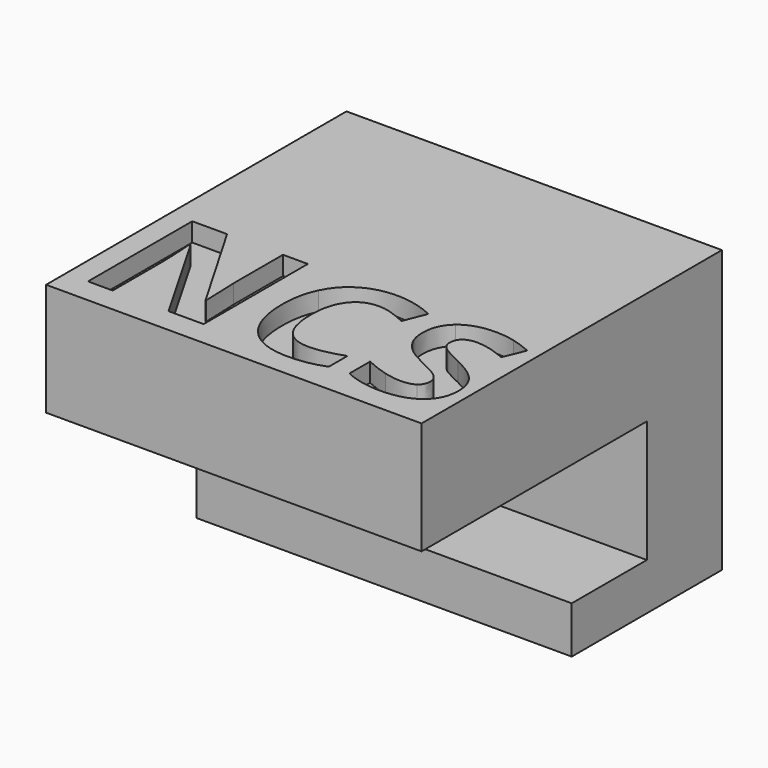
from build123d import *

# Parameters (mm, degrees)
F0_W         = 40
F0_H         = 10
F1_DEPTH     = 5
F2_DEPTH     = 13
F3_START     = 13
F0_H_2       = 20
F3_DEPTH     = 12
F4_START     = 13
F0_TEXT_SIZE = 19.4444444444
F4_DEPTH     = 10


# Not quite as in the source:
# - Text() gives the source's letters only with a copy of the font that has no kerning and outlines rounded to 1/6400 em; it was checked with that copy


with BuildPart() as f1:
    # F0 (on Top) → F1 (new body)
    with BuildSketch(Plane.XY):
        with Locations((0, 15)):
            Rectangle(F0_W, F0_H)
        with Locations((0, 5)):
            Rectangle(F0_W, F0_H)
    extrude(amount=-F1_DEPTH)

    # F0 (on Top) → F2 (join)
    with BuildSketch(Plane.XY):
        with Locations((0, 15)):
            Rectangle(F0_W, F0_H)
    extrude(amount=F2_DEPTH)

    # F0 (on Top) → F3 (join)
    with BuildSketch(Plane.XY.offset(F3_START)):
        with Locations((0, -10)):
            Rectangle(F0_W, F0_H_2)
        with BuildLine():
            Line((-5.3385416667, -3.4717519035), (-5.3385416667, -17.3532623202))
            Line((-5.3385416667, -17.3532623202), (-9.0785590278, -17.3532623202))
            Line((-9.0785590278, -17.3532623202), (-15.1184895833, -6.8532623202))
            Line((-15.1184895833, -6.8532623202), (-15.2035590278, -6.8532623202))
            add(Edge.make_bspline(
                [(-15.2035590278, -6.8532623202), (-15.0212673611, -9.6332102368), (-15.0212673611, -10.8211442646)],
                knots=[0, 0, 0, 1, 1, 1], degree=2))
            Line((-15.0212673611, -10.8211442646), (-15.0212673611, -17.3532623202))
            Line((-15.0212673611, -17.3532623202), (-17.65234375, -17.3532623202))
            Line((-17.65234375, -17.3532623202), (-17.65234375, -3.4717519035))
            Line((-17.65234375, -3.4717519035), (-13.9396701389, -3.4717519035))
            Line((-13.9396701389, -3.4717519035), (-7.9118923611, -13.8684532924))
            Line((-7.9118923611, -13.8684532924), (-7.8450520833, -13.8684532924))
            add(Edge.make_bspline(
                [(-7.8450520833, -13.8684532924), (-7.9878472222, -11.1614220424), (-7.9878472222, -10.0433664868)],
                knots=[0, 0, 0, 1, 1, 1], degree=2))
            Line((-7.9878472222, -10.0433664868), (-7.9878472222, -3.4717519035))
            Line((-7.9878472222, -3.4717519035), (-5.3385416667, -3.4717519035))
        make_face(mode=Mode.SUBTRACT)
        with BuildLine():
            add(Edge.make_bspline(
                [(5.5989583333, -5.998010584), (4.8120659722, -5.7230539868), (4.0525173611, -5.7230539868)],
                knots=[0, 0, 0, 1, 1, 1], degree=2))
            add(Edge.make_bspline(
                [(4.0525173611, -5.7230539868), (2.390625, -5.7230539868), (1.4791666667, -6.9717519035)],
                knots=[0, 0, 0, 1, 1, 1], degree=2))
            add(Edge.make_bspline(
                [(1.4791666667, -6.9717519035), (0.5677083333, -8.2204498202), (0.5677083333, -10.4504845424)],
                knots=[0, 0, 0, 1, 1, 1], degree=2))
            add(Edge.make_bspline(
                [(0.5677083333, -10.4504845424), (0.5677083333, -15.0928456535), (4.0525173611, -15.0928456535)],
                knots=[0, 0, 0, 1, 1, 1], degree=2))
            add(Edge.make_bspline(
                [(4.0525173611, -15.0928456535), (5.5138888889, -15.0928456535), (7.5920138889, -14.3636789868)],
                knots=[0, 0, 0, 1, 1, 1], degree=2))
            Line((7.5920138889, -14.3636789868), (7.5920138889, -16.8306928757))
            add(Edge.make_bspline(
                [(7.5920138889, -16.8306928757), (5.8845486111, -17.5446685702), (3.7760416667, -17.5446685702)],
                knots=[0, 0, 0, 1, 1, 1], degree=2))
            add(Edge.make_bspline(
                [(3.7760416667, -17.5446685702), (0.7469618056, -17.5446685702), (-0.8572048611, -15.7065609313)],
                knots=[0, 0, 0, 1, 1, 1], degree=2))
            add(Edge.make_bspline(
                [(-0.8572048611, -15.7065609313), (-2.4613715278, -13.8684532924), (-2.4613715278, -10.4322553757)],
                knots=[0, 0, 0, 1, 1, 1], degree=2))
            add(Edge.make_bspline(
                [(-2.4613715278, -10.4322553757), (-2.4613715278, -8.2660227368), (-1.6729600694, -6.6375505146)],
                knots=[0, 0, 0, 1, 1, 1], degree=2))
            add(Edge.make_bspline(
                [(-1.6729600694, -6.6375505146), (-0.8845486111, -5.0090782924), (0.5920138889, -4.1416737785)],
                knots=[0, 0, 0, 1, 1, 1], degree=2))
            add(Edge.make_bspline(
                [(0.5920138889, -4.1416737785), (2.0685763889, -3.2742692646), (4.0525173611, -3.2742692646)],
                knots=[0, 0, 0, 1, 1, 1], degree=2))
            add(Edge.make_bspline(
                [(4.0525173611, -3.2742692646), (6.0729166667, -3.2742692646), (8.1145833333, -4.2495296813)],
                knots=[0, 0, 0, 1, 1, 1], degree=2))
            Line((8.1145833333, -4.2495296813), (7.1666666667, -6.6436269035))
            add(Edge.make_bspline(
                [(7.1666666667, -6.6436269035), (6.3858506944, -6.2729671813), (5.5989583333, -5.998010584)],
                knots=[0, 0, 0, 1, 1, 1], degree=2))
        make_face(mode=Mode.SUBTRACT)
        with BuildLine():
            add(Edge.make_bspline(
                [(18.017578125, -11.2054758618), (18.7391493056, -12.1397206535), (18.7391493056, -13.4977935702)],
                knots=[0, 0, 0, 1, 1, 1], degree=2))
            add(Edge.make_bspline(
                [(18.7391493056, -13.4977935702), (18.7391493056, -15.3784359313), (17.3856336806, -16.4615522507)],
                knots=[0, 0, 0, 1, 1, 1], degree=2))
            add(Edge.make_bspline(
                [(17.3856336806, -16.4615522507), (16.0321180556, -17.5446685702), (13.6228298611, -17.5446685702)],
                knots=[0, 0, 0, 1, 1, 1], degree=2))
            add(Edge.make_bspline(
                [(13.6228298611, -17.5446685702), (11.3988715278, -17.5446685702), (9.69140625, -16.7061269035)],
                knots=[0, 0, 0, 1, 1, 1], degree=2))
            Line((9.69140625, -16.7061269035), (9.69140625, -13.9717519035))
            add(Edge.make_bspline(
                [(9.69140625, -13.9717519035), (11.0950520833, -14.6006581535), (12.0687934028, -14.8558664868)],
                knots=[0, 0, 0, 1, 1, 1], degree=2))
            add(Edge.make_bspline(
                [(12.0687934028, -14.8558664868), (13.0425347222, -15.1110748202), (13.8506944444, -15.1110748202)],
                knots=[0, 0, 0, 1, 1, 1], degree=2))
            add(Edge.make_bspline(
                [(13.8506944444, -15.1110748202), (14.8168402778, -15.1110748202), (15.3348524306, -14.7419341952)],
                knots=[0, 0, 0, 1, 1, 1], degree=2))
            add(Edge.make_bspline(
                [(15.3348524306, -14.7419341952), (15.8528645833, -14.3727935702), (15.8528645833, -13.640588709)],
                knots=[0, 0, 0, 1, 1, 1], degree=2))
            add(Edge.make_bspline(
                [(15.8528645833, -13.640588709), (15.8528645833, -13.2334706535), (15.625, -12.9144602368)],
                knots=[0, 0, 0, 1, 1, 1], degree=2))
            add(Edge.make_bspline(
                [(15.625, -12.9144602368), (15.3971354167, -12.5954498202), (14.955078125, -12.3022640563)],
                knots=[0, 0, 0, 1, 1, 1], degree=2))
            add(Edge.make_bspline(
                [(14.955078125, -12.3022640563), (14.5130208333, -12.0090782924), (13.1549479167, -11.3619428757)],
                knots=[0, 0, 0, 1, 1, 1], degree=2))
            add(Edge.make_bspline(
                [(13.1549479167, -11.3619428757), (11.8849826389, -10.7634185702), (11.2484809028, -10.2135053757)],
                knots=[0, 0, 0, 1, 1, 1], degree=2))
            add(Edge.make_bspline(
                [(11.2484809028, -10.2135053757), (10.6119791667, -9.6635921813), (10.2322048611, -8.9313873202)],
                knots=[0, 0, 0, 1, 1, 1], degree=2))
            add(Edge.make_bspline(
                [(10.2322048611, -8.9313873202), (9.8524305556, -8.199182459), (9.8524305556, -7.2239220424)],
                knots=[0, 0, 0, 1, 1, 1], degree=2))
            add(Edge.make_bspline(
                [(9.8524305556, -7.2239220424), (9.8524305556, -5.3797380146), (11.1011284722, -4.3270036396)],
                knots=[0, 0, 0, 1, 1, 1], degree=2))
            add(Edge.make_bspline(
                [(11.1011284722, -4.3270036396), (12.3498263889, -3.2742692646), (14.5525173611, -3.2742692646)],
                knots=[0, 0, 0, 1, 1, 1], degree=2))
            add(Edge.make_bspline(
                [(14.5525173611, -3.2742692646), (15.6341145833, -3.2742692646), (16.6169704861, -3.5294775979)],
                knots=[0, 0, 0, 1, 1, 1], degree=2))
            add(Edge.make_bspline(
                [(16.6169704861, -3.5294775979), (17.5998263889, -3.7846859313), (18.6723090278, -4.2495296813)],
                knots=[0, 0, 0, 1, 1, 1], degree=2))
            Line((18.6723090278, -4.2495296813), (17.7243923611, -6.5403282924))
            add(Edge.make_bspline(
                [(17.7243923611, -6.5403282924), (16.6124131944, -6.0845991257), (15.8862847222, -5.9038265563)],
                knots=[0, 0, 0, 1, 1, 1], degree=2))
            add(Edge.make_bspline(
                [(15.8862847222, -5.9038265563), (15.16015625, -5.7230539868), (14.4583333333, -5.7230539868)],
                knots=[0, 0, 0, 1, 1, 1], degree=2))
            add(Edge.make_bspline(
                [(14.4583333333, -5.7230539868), (13.6228298611, -5.7230539868), (13.1762152778, -6.1119428757)],
                knots=[0, 0, 0, 1, 1, 1], degree=2))
            add(Edge.make_bspline(
                [(13.1762152778, -6.1119428757), (12.7296006944, -6.5008317646), (12.7296006944, -7.1266998202)],
                knots=[0, 0, 0, 1, 1, 1], degree=2))
            add(Edge.make_bspline(
                [(12.7296006944, -7.1266998202), (12.7296006944, -7.515588709), (12.9103732639, -7.8057362785)],
                knots=[0, 0, 0, 1, 1, 1], degree=2))
            add(Edge.make_bspline(
                [(12.9103732639, -7.8057362785), (13.0911458333, -8.0958838479), (13.4845920139, -8.3662831535)],
                knots=[0, 0, 0, 1, 1, 1], degree=2))
            add(Edge.make_bspline(
                [(13.4845920139, -8.3662831535), (13.8780381944, -8.636682459), (15.3485243056, -9.3385053757)],
                knots=[0, 0, 0, 1, 1, 1], degree=2))
            add(Edge.make_bspline(
                [(15.3485243056, -9.3385053757), (17.2960069444, -10.2712310702), (18.017578125, -11.2054758618)],
                knots=[0, 0, 0, 1, 1, 1], degree=2))
        make_face(mode=Mode.SUBTRACT)
        with Locations((0, 5)):
            Rectangle(F0_W, F0_H)
        with Locations((0, 15)):
            Rectangle(F0_W, F0_H)
    extrude(amount=F3_DEPTH)

    # F0 (on Top) → F4 (join)
    with BuildSketch(Plane.XY.offset(F4_START)):
        with Locations((-19.3993055556, -17.3532623202)):
            Text('NCS', F0_TEXT_SIZE, font='Open Sans', font_style=FontStyle.BOLD, text_align=(TextAlign.LEFT, TextAlign.BOTTOM))
    extrude(amount=F4_DEPTH)


solid = f1.part
